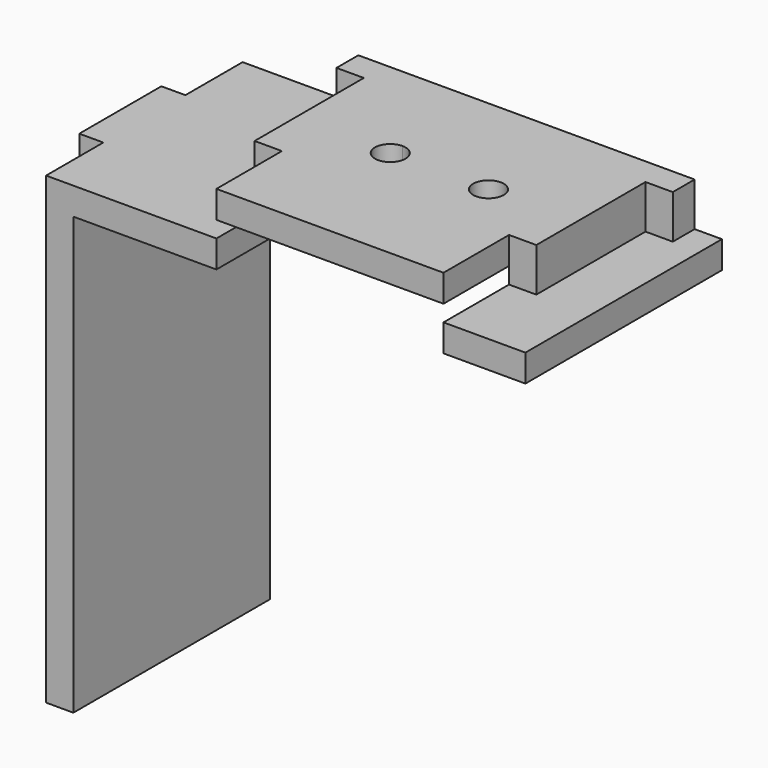
from build123d import *

# Parameters (mm, degrees)
F1_DEPTH       = 6.35
F2_W           = 26.416
F2_H           = 3.175
F3_DEPTH       = 22.225
F4_W           = 3.175
F4_H           = 19.05
F5_DEPTH       = 8.255
F6_W           = 3.175
F6_H           = 3.175
F7_DEPTH       = 9.525
F8_W           = 3.175
F8_H           = 3.175
F9_DEPTH       = 9.525
F10_W          = 28.575
F10_H          = 3.175
F11_DEPTH      = 13.462
F12_W          = 3.175
F12_H          = 28.575
F13_DEPTH      = 50.8
F13_DEPTH_BACK = 3.175
F15_DEPTH      = 2.794
F17_DEPTH      = 25.4
F18_W          = 3.175
F18_H          = 3.175
F19_DEPTH      = 5.08
F20_W          = 28.575
F20_H          = 3.175
F21_DEPTH      = 6.35
F22_W          = 3.175
F22_H          = 3.175
F23_DEPTH      = 5.08


with BuildPart() as f1:
    # F0 (on Front) → F1 (new body)
    with BuildSketch(Plane.XZ):
        Polygon((0, 2.54), (0, 0), (3.175, 0), (6.35, 0), (6.35, 5.08), (6.35, 8.255), (-20.066, 8.255), (-20.066, 5.08), (-20.066, 0), (-16.891, 0), (-13.716, 0), (-13.716, 2.54), (-16.891, 2.54), (-16.891, 5.08), (3.175, 5.08), (3.175, 2.54), align=None)
    extrude(amount=F1_DEPTH)

    # F2 (on face) → F3 (join)
    with BuildSketch(Plane.XZ.offset(6.35)):
        with Locations((-6.858, 6.6675)):
            Rectangle(F2_W, F2_H)
    extrude(amount=F3_DEPTH)

    # F4 (on face) → F5 (join, through all)
    with BuildSketch(Plane.XY.offset(8.255)):
        with Locations((-21.6535, -9.525)):
            Rectangle(F4_W, F4_H)
        with Locations((7.9375, -9.525)):
            Rectangle(F4_W, F4_H)
    extrude(amount=-F5_DEPTH)

    # F6 (on face) → F7 (join, through all)
    with BuildSketch(Plane.XZ.offset(19.05)):
        with Locations((-21.6535, 1.5875)):
            Rectangle(F6_W, F6_H)
    extrude(amount=F7_DEPTH)

    # F8 (on face) → F9 (join, through all)
    with BuildSketch(Plane.XZ.offset(19.05)):
        with Locations((7.9375, 1.5875)):
            Rectangle(F8_W, F8_H)
    extrude(amount=F9_DEPTH)

    # F10 (on face) → F11 (join)
    with BuildSketch(Plane(origin=(-23.241, 0, 0), x_dir=(0, -1, 0), z_dir=(-1, 0, 0))):
        with Locations((14.2875, 1.5875)):
            Rectangle(F10_W, F10_H)
    extrude(amount=F11_DEPTH)

    # F12 (on face) → F13 (join, two sides)
    with BuildSketch(Plane(origin=(0, 0, 0), x_dir=(1, 0, 0), z_dir=(0, 0, -1))) as f13_sk:
        with Locations((-38.2905, 14.2875)):
            Rectangle(F12_W, F12_H)
    extrude(amount=F13_DEPTH)
    extrude(f13_sk.sketch, amount=-F13_DEPTH_BACK)

    # F14 (on face) → F15 (join)
    with BuildSketch(Plane(origin=(-39.878, 0, 0), x_dir=(0, -1, 0), z_dir=(-1, 0, 0))):
        Polygon((20.2565, 3.175), (14.2875, 3.175), (8.3185, 3.175), (8.3185, -21.463), (20.2565, -21.463), align=None)
    extrude(amount=F15_DEPTH)

    # F16 (on face) → F17 (cut)
    with BuildSketch(Plane.XY.offset(8.255)):
        with BuildLine():
            ThreePointArc((-10.361326316, -13.208), (-10.882090459, -11.9507641431), (-12.139326316, -11.43))
            Line((-12.139326316, -11.43), (-12.139326316, -13.208))
            Line((-12.139326316, -13.208), (-10.361326316, -13.208))
        make_face()
        with BuildLine():
            ThreePointArc((1.068673684, -13.208), (-0.709326316, -11.43), (-2.487326316, -13.208))
            ThreePointArc((-2.487326316, -13.208), (-0.709326316, -14.986), (1.068673684, -13.208))
        make_face()
        with BuildLine():
            Line((-12.139326316, -13.208), (-12.139326316, -11.43))
            ThreePointArc((-12.139326316, -11.43), (-13.3965621729, -14.4652358569), (-10.361326316, -13.208))
            Line((-10.361326316, -13.208), (-12.139326316, -13.208))
        make_face()
    extrude(amount=-F17_DEPTH, mode=Mode.SUBTRACT)

    # F18 (on face) → F19 (join, through all)
    with BuildSketch(Plane.XY.offset(3.175)):
        with Locations((-24.8285, -1.5875)):
            Rectangle(F18_W, F18_H)
    extrude(amount=F19_DEPTH)

    # F20 (on face) → F21 (join)
    with BuildSketch(Plane.YZ.offset(9.525)):
        with Locations((-14.2875, 1.5875)):
            Rectangle(F20_W, F20_H)
    extrude(amount=F21_DEPTH)

    # F22 (on face) → F23 (join, through all)
    with BuildSketch(Plane.XY.offset(3.175)):
        with Locations((11.1125, -1.5875)):
            Rectangle(F22_W, F22_H)
    extrude(amount=F23_DEPTH)


solid = f1.part
